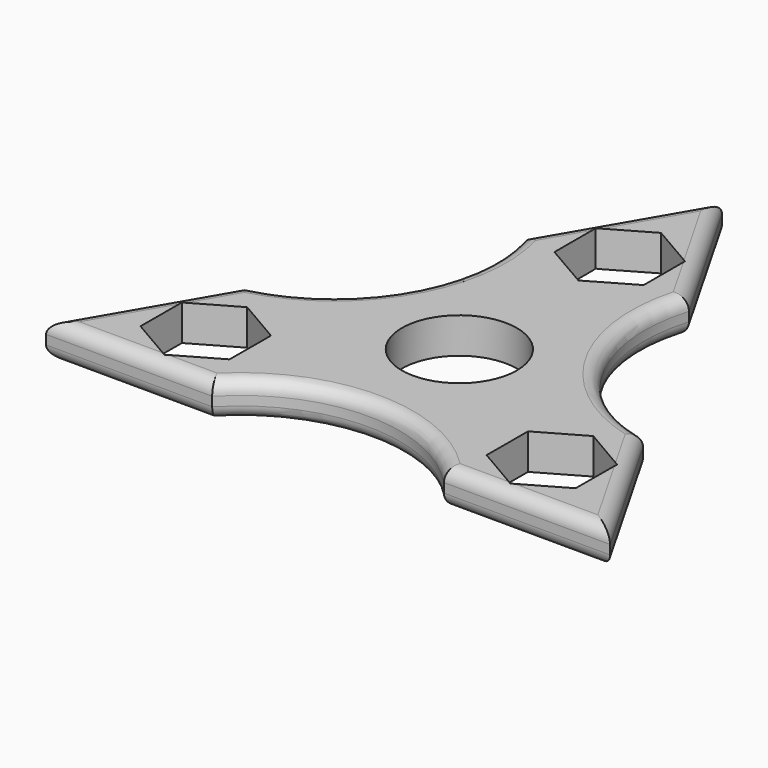
from build123d import *

# Parameters (mm, degrees)
F0_R         = 11.049
F1_DEPTH     = 6.858
F2_DEPTH     = 46.99
F3_DEPTH     = 37.592
F4_DEPTH     = 42.418
F5_DEPTH     = 29.718
F6_DEPTH     = 25.4
F7_T1_DEPTH  = 44.7190403061
F7_T3_DEPTH  = 44.7190403061
F7_T5_DEPTH  = 44.7190403061
F7_T7_DEPTH  = 44.7190403061
F7_T9_DEPTH  = 44.7190403061
F7_T11_DEPTH = 44.7190403061
F7_T14_ANGLE = 117.6067451319
F7_T16_ANGLE = 117.3898443425
F7_T18_ANGLE = 118.1021999746
F7_T20_ANGLE = 118.1021999746
F7_T22_ANGLE = 117.3898443425
F7_T24_ANGLE = 117.6067451319


# Not quite as in the source:
# - a fillet or chamfer that OpenCascade refuses, or shapes differently, is made with other operations: its cross-section is extruded or revolved along the edge and cut away or added


with BuildPart() as f1:
    # F0 (on Top) → F1 (new body)
    with BuildSketch(Plane.XY):
        with BuildLine():
            Line((22.208523276, -31.466120161), (54.2273194105, -31.5911650137))
            Line((54.2273194105, -31.5911650137), (38.3262133623, -3.7995517362))
            ThreePointArc((38.3262133623, -3.7995517362), (18.8280371905, 10.7725526064), (16.14619778, 34.966205418))
            Line((16.14619778, 34.966205418), (0.2450917317, 62.7578186955))
            Line((0.2450917317, 62.7578186955), (-15.8725983546, 35.0912502707))
            ThreePointArc((-15.8725983546, 35.0912502707), (-18.7017871859, 10.8950848293), (-38.354721056, -3.500085257))
            Line((-38.354721056, -3.500085257), (-54.4724111423, -31.1666536818))
            Line((-54.4724111423, -31.1666536818), (-22.4536150077, -31.2916985345))
            ThreePointArc((-22.4536150077, -31.2916985345), (-0.0847964289, -21.7128455258), (22.208523276, -31.466120161))
        make_face()
        Polygon((-41.9885712831, -14.1401743102), (-33.3904459647, -9.2207152943), (-24.8310068248, -14.207180737), (-24.8696930034, -24.1131051956), (-33.4678183218, -29.0325642115), (-42.0272574616, -24.0460987688), align=None, mode=Mode.SUBTRACT)
        Polygon((24.6805966683, -24.3066168019), (24.7192828468, -14.4006923433), (33.3174081652, -9.4812333274), (41.8768473051, -14.4676987701), (41.8381611265, -24.3736232287), (33.2400358081, -29.2930822446), align=None, mode=Mode.SUBTRACT)
        Circle(F0_R, mode=Mode.SUBTRACT)
        Polygon((-8.5839493951, 33.5699382512), (-8.5737367865, 43.4759329869), (0.0102126086, 48.4200859762), (8.5839493951, 43.4582442299), (8.5737367865, 33.5522494943), (-0.0102126086, 28.6080965049), align=None, mode=Mode.SUBTRACT)
        with BuildLine():
            Line((-22.4536150077, -31.2916985345), (22.208523276, -31.466120161))
            ThreePointArc((22.208523276, -31.466120161), (-0.0847964289, -21.7128455258), (-22.4536150077, -31.2916985345))
        make_face()
        with BuildLine():
            ThreePointArc((16.14619778, 34.966205418), (18.8280371905, 10.7725526064), (38.3262133623, -3.7995517362))
            Line((38.3262133623, -3.7995517362), (16.14619778, 34.966205418))
        make_face()
        with BuildLine():
            Line((-15.8725983546, 35.0912502707), (-38.354721056, -3.500085257))
            ThreePointArc((-38.354721056, -3.500085257), (-18.7017871859, 10.8950848293), (-15.8725983546, 35.0912502707))
        make_face()
    extrude(amount=F1_DEPTH)

    # F0 (on Top) → F2 (cut)
    with BuildSketch(Plane.XY):
        with BuildLine():
            Line((-15.8725983546, 35.0912502707), (-38.354721056, -3.500085257))
            ThreePointArc((-38.354721056, -3.500085257), (-18.7017871859, 10.8950848293), (-15.8725983546, 35.0912502707))
        make_face()
    extrude(amount=F2_DEPTH, mode=Mode.SUBTRACT)

    # F0 (on Top) → F3 (cut)
    with BuildSketch(Plane.XY):
        with BuildLine():
            Line((-22.4536150077, -31.2916985345), (22.208523276, -31.466120161))
            ThreePointArc((22.208523276, -31.466120161), (-0.0847964289, -21.7128455258), (-22.4536150077, -31.2916985345))
        make_face()
    extrude(amount=F3_DEPTH, mode=Mode.SUBTRACT)

    # F0 (on Top) → F4 (cut)
    with BuildSketch(Plane.XY):
        with BuildLine():
            ThreePointArc((16.14619778, 34.966205418), (18.8280371905, 10.7725526064), (38.3262133623, -3.7995517362))
            Line((38.3262133623, -3.7995517362), (16.14619778, 34.966205418))
        make_face()
    extrude(amount=F4_DEPTH, mode=Mode.SUBTRACT)

    # F0 (on Top) → F5 (cut)
    with BuildSketch(Plane.XY):
        Circle(F0_R)
    extrude(amount=F5_DEPTH, mode=Mode.SUBTRACT)

    # F0 (on Top) → F6 (cut)
    with BuildSketch(Plane.XY):
        Circle(F0_R)
    extrude(amount=F6_DEPTH, mode=Mode.SUBTRACT)

    # F7: fillet of radius 2.54 on 18 edges, made by hand

    # F7_s2 → F7_t1 (cut)
    with BuildSketch(Plane(origin=(-7.936508422, 13.8712597833, 0), x_dir=(0, 0, 1), z_dir=(-0.4966140739, 0.8679714636, 0))):
        with BuildLine():
            ThreePointArc((0, 28.8391486396), (0.7439487758, 30.6351998638), (2.54, 31.3791486396))
            Line((2.54, 31.3791486396), (0, 31.3791486396))
            Line((0, 31.3791486396), (0, 28.8391486396))
        make_face()
        with BuildLine():
            ThreePointArc((6.858, 28.8391486396), (6.1140512242, 30.6351998638), (4.318, 31.3791486396))
            Line((4.318, 31.3791486396), (6.858, 31.3791486396))
            Line((6.858, 31.3791486396), (6.858, 28.8391486396))
        make_face()
    extrude(amount=F7_T1_DEPTH, mode=Mode.SUBTRACT)

    # F7_s4 → F7_t3 (cut)
    with BuildSketch(Plane(origin=(30.1446132086, -52.6861106484, 0), x_dir=(0, 0, 1), z_dir=(-0.4966140739, 0.8679714636, 0))):
        with BuildLine():
            ThreePointArc((2.54, 31.3791486396), (0.7439487758, 30.6351998638), (0, 28.8391486396))
            Line((0, 28.8391486396), (0, 31.3791486396))
            Line((0, 31.3791486396), (2.54, 31.3791486396))
        make_face()
        with BuildLine():
            ThreePointArc((4.318, 31.3791486396), (6.1140512242, 30.6351998638), (6.858, 28.8391486396))
            Line((6.858, 28.8391486396), (6.858, 31.3791486396))
            Line((6.858, 31.3791486396), (4.318, 31.3791486396))
        make_face()
    extrude(amount=F7_T3_DEPTH, mode=Mode.SUBTRACT)

    # F7_s6 → F7_t5 (cut)
    with BuildSketch(Plane(origin=(15.9811175658, -0.0624119809, 0), x_dir=(0, 0, 1), z_dir=(0.9999923742, -0.0039053279, 0))):
        with BuildLine():
            ThreePointArc((0, 28.8391486396), (0.7439487758, 30.6351998638), (2.54, 31.3791486396))
            Line((2.54, 31.3791486396), (0, 31.3791486396))
            Line((0, 31.3791486396), (0, 28.8391486396))
        make_face()
        with BuildLine():
            ThreePointArc((6.858, 28.8391486396), (6.1140512242, 30.6351998638), (4.318, 31.3791486396))
            Line((4.318, 31.3791486396), (6.858, 31.3791486396))
            Line((6.858, 31.3791486396), (6.858, 28.8391486396))
        make_face()
    extrude(amount=F7_T5_DEPTH, mode=Mode.SUBTRACT)

    # F7_s8 → F7_t7 (cut)
    with BuildSketch(Plane(origin=(-8.0446091438, -13.8088478024, 0), x_dir=(0, 0, 1), z_dir=(-0.5033783003, -0.8640661357, 0))):
        with BuildLine():
            ThreePointArc((0, 28.8391486396), (0.7439487758, 30.6351998638), (2.54, 31.3791486396))
            Line((2.54, 31.3791486396), (0, 31.3791486396))
            Line((0, 31.3791486396), (0, 28.8391486396))
        make_face()
        with BuildLine():
            ThreePointArc((6.858, 28.8391486396), (6.1140512242, 30.6351998638), (4.318, 31.3791486396))
            Line((4.318, 31.3791486396), (6.858, 31.3791486396))
            Line((6.858, 31.3791486396), (6.858, 28.8391486396))
        make_face()
    extrude(amount=F7_T7_DEPTH, mode=Mode.SUBTRACT)

    # F7_s10 → F7_t9 (cut)
    with BuildSketch(Plane(origin=(-60.6998168524, 0.2370544983, 0), x_dir=(0, 0, 1), z_dir=(0.9999923742, -0.0039053279, 0))):
        with BuildLine():
            ThreePointArc((0, 28.8391486396), (0.7439487758, 30.6351998638), (2.54, 31.3791486396))
            Line((2.54, 31.3791486396), (0, 31.3791486396))
            Line((0, 31.3791486396), (0, 28.8391486396))
        make_face()
        with BuildLine():
            ThreePointArc((6.858, 28.8391486396), (6.1140512242, 30.6351998638), (4.318, 31.3791486396))
            Line((4.318, 31.3791486396), (6.858, 31.3791486396))
            Line((6.858, 31.3791486396), (6.858, 28.8391486396))
        make_face()
    extrude(amount=F7_T9_DEPTH, mode=Mode.SUBTRACT)

    # F7_s12 → F7_t11 (cut)
    with BuildSketch(Plane(origin=(30.5552036438, 52.4490561501, 0), x_dir=(0, 0, 1), z_dir=(-0.5033783003, -0.8640661357, 0))):
        with BuildLine():
            ThreePointArc((0, 28.8391486396), (0.7439487758, 30.6351998638), (2.54, 31.3791486396))
            Line((2.54, 31.3791486396), (0, 31.3791486396))
            Line((0, 31.3791486396), (0, 28.8391486396))
        make_face()
        with BuildLine():
            ThreePointArc((6.858, 28.8391486396), (6.1140512242, 30.6351998638), (4.318, 31.3791486396))
            Line((4.318, 31.3791486396), (6.858, 31.3791486396))
            Line((6.858, 31.3791486396), (6.858, 28.8391486396))
        make_face()
    extrude(amount=F7_T11_DEPTH, mode=Mode.SUBTRACT)

    # F7_s13 → F7_t14 (revolve, cut)
    with BuildSketch(Plane(origin=(21.6971694487, 39.0990533159, 0), x_dir=(0, 0, 1), z_dir=(0.4852237348, 0.8743900315, 0))):
        with BuildLine():
            ThreePointArc((0, -6.0457943644), (0.7439487758, -4.2497431402), (2.54, -3.5057943644))
            Line((2.54, -3.5057943644), (0, -3.5057943644))
            Line((0, -3.5057943644), (0, -6.0457943644))
        make_face()
    revolve(axis=Axis((45.3732523459, 25.9605259365, 0), (0, 0, 1)), revolution_arc=F7_T14_ANGLE, mode=Mode.SUBTRACT)

    # F7_s15 → F7_t16 (revolve, cut)
    with BuildSketch(Plane(origin=(23.0875297384, -38.3008650951, 0), x_dir=(0, 0, 1), z_dir=(0.5162541117, -0.8564354571, 0))):
        with BuildLine():
            ThreePointArc((0, -5.9721181992), (0.7439487758, -4.176066975), (2.54, -3.4321181992))
            Line((2.54, -3.4321181992), (0, -3.4321181992))
            Line((0, -3.4321181992), (0, -5.9721181992))
        make_face()
    revolve(axis=Axis((-0.2044107419, -52.3411058879, 0), (0, 0, 1)), revolution_arc=F7_T16_ANGLE, mode=Mode.SUBTRACT)

    # F7_s17 → F7_t18 (revolve, cut)
    with BuildSketch(Plane(origin=(-44.6992655412, -0.5657482073, 0), x_dir=(0, 0, 1), z_dir=(-0.9999199127, -0.0126557538, 0))):
        with BuildLine():
            ThreePointArc((0, -6.2140449518), (0.7439487758, -4.4179937276), (2.54, -3.6740449518))
            Line((2.54, -3.6740449518), (0, -3.6740449518))
            Line((0, -3.6740449518), (0, -6.2140449518))
        make_face()
    revolve(axis=Axis((-45.0385149903, 26.2380507555, 0), (0, 0, 1)), revolution_arc=F7_T18_ANGLE, mode=Mode.SUBTRACT)

    # F7_s19 → F7_t20 (revolve, cut)
    with BuildSketch(Plane(origin=(-21.5544505992, 39.1631213047, 0), x_dir=(0, 0, 1), z_dir=(-0.4821717785, 0.8760766953, 0))):
        with BuildLine():
            ThreePointArc((6.858, 6.2140449518), (6.1140512242, 4.4179937276), (4.318, 3.6740449518))
            Line((4.318, 3.6740449518), (6.858, 3.6740449518))
            Line((6.858, 3.6740449518), (6.858, 6.2140449518))
        make_face()
    revolve(axis=Axis((-45.0385149903, 26.2380507555, 6.858), (0, 0, -1)), revolution_arc=F7_T20_ANGLE, mode=Mode.SUBTRACT)

    # F7_s21 → F7_t22 (revolve, cut)
    with BuildSketch(Plane(origin=(-23.3859780913, -38.1193694225, 0), x_dir=(0, 0, 1), z_dir=(-0.5229276359, -0.8523770807, 0))):
        with BuildLine():
            ThreePointArc((6.858, 5.9721181992), (6.1140512242, 4.176066975), (4.318, 3.4321181992))
            Line((4.318, 3.4321181992), (6.858, 3.4321181992))
            Line((6.858, 3.4321181992), (6.858, 5.9721181992))
        make_face()
    revolve(axis=Axis((-0.2044107419, -52.3411058879, 6.858), (0, 0, -1)), revolution_arc=F7_T22_ANGLE, mode=Mode.SUBTRACT)

    # F7_s23 → F7_t24 (revolve, cut)
    with BuildSketch(Plane(origin=(44.7020643692, -1.1084103144, 0), x_dir=(0, 0, 1), z_dir=(0.9996927331, -0.0247878874, 0))):
        with BuildLine():
            ThreePointArc((4.318, 3.5057943644), (6.1140512242, 4.2497431402), (6.858, 6.0457943644))
            Line((6.858, 6.0457943644), (6.858, 3.5057943644))
            Line((6.858, 3.5057943644), (4.318, 3.5057943644))
        make_face()
    revolve(axis=Axis((45.3732523459, 25.9605259365, 6.858), (0, 0, -1)), revolution_arc=F7_T24_ANGLE, mode=Mode.SUBTRACT)


solid = f1.part
